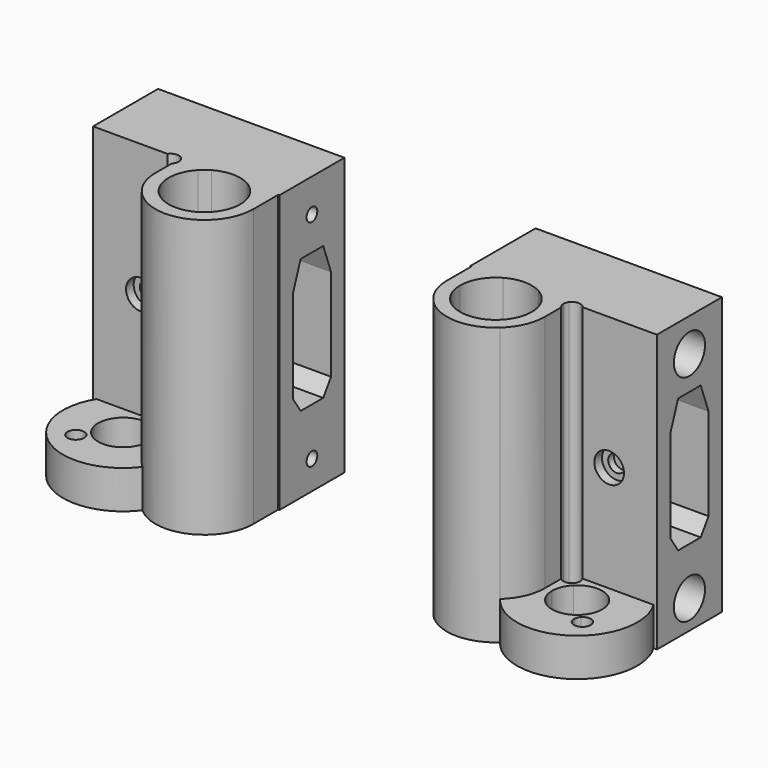
from build123d import *
from build123d import SkipClean  # not in build123d's __all__

# Parameters (mm, degrees)
F0_W           = 39
F0_H           = 58
F1_DEPTH       = 17
F3_DEPTH       = 58.001
F4_DEPTH       = 58
F5_DEPTH       = 8
F7_DEPTH       = 39.001
F6_R           = 4.075
F8_DEPTH       = 19.6
F10_R          = 1.4
F9_R           = 1.4
F11_DEPTH      = 19.401
F12_R          = 1.8
F13_DEPTH      = 3.501
F13_DEPTH_BACK = 32.601
F14_R          = 3.1
F14_R_2        = 1.8
F15_DEPTH      = 2
F16_R          = 1.8
F17_DEPTH      = 2


# Not quite as in the source:
# - a feature names something its author has since deleted; it is built from what else it names


with BuildPart() as f1:
    # F0 (on Front) → F1 (new body)
    with BuildSketch(Plane.XZ):
        with Locations((-21.25, -2)):
            Rectangle(F0_W, F0_H)
    extrude(amount=F1_DEPTH)

    # F2 (on face) → F3 (cut, through all)
    with BuildSketch(Plane(origin=(0, 0, -31), x_dir=(1, 0, 0), z_dir=(0, 0, -1))):
        with BuildLine():
            ThreePointArc((-15.9786113032, 17), (-12.25, 16.0065), (-8.5213886968, 17))
            Line((-8.5213886968, 17), (-15.9786113032, 17))
        make_face()
        with BuildLine():
            ThreePointArc((-25.186178146, 17), (-23.7501234559, 16.2501234559), (-22.3140687659, 17))
            Line((-22.3140687659, 17), (-22.5, 17))
            Line((-22.5, 17), (-25.186178146, 17))
        make_face()
        with BuildLine():
            Line((-22.5, 17), (-22.3140687659, 17))
            ThreePointArc((-22.3140687659, 17), (-22.0804534724, 17.4760031013), (-22.0001234559, 18.0001234559))
            ThreePointArc((-22.0001234559, 18.0001234559), (-22.1299049448, 18.6614796202), (-22.5, 19.2247423129))
            Line((-22.5, 19.2247423129), (-22.5, 17))
        make_face()
    extrude(amount=-F3_DEPTH, mode=Mode.SUBTRACT)

    # F2 (on face) → F4 (join, through all)
    with BuildSketch(Plane(origin=(0, 0, -31), x_dir=(1, 0, 0), z_dir=(0, 0, -1))):
        with BuildLine():
            ThreePointArc((-15.9786113032, 17), (-16.907616188, 17.6298080359), (-17.7321335956, 18.3913060876))
            ThreePointArc((-17.7321335956, 18.3913060876), (-18.0724084231, 17.6843790924), (-18.4560201964, 17))
            Line((-18.4560201964, 17), (-15.9786113032, 17))
        make_face()
        with BuildLine():
            ThreePointArc((-17.7321335956, 18.3913060876), (-19.7435, 23.5), (-17.7321335956, 28.6086939124))
            ThreePointArc((-17.7321335956, 28.6086939124), (-18.382014032, 29.8754906477), (-19.1706617647, 31.0608822725))
            ThreePointArc((-19.1706617647, 31.0608822725), (-21.6308124139, 27.6307212997), (-22.5, 23.5))
            Line((-22.5, 23.5), (-22.5, 19.2247423129))
            ThreePointArc((-22.5, 19.2247423129), (-22.1299049448, 18.6614796202), (-22.0001234559, 18.0001234559))
            ThreePointArc((-22.0001234559, 18.0001234559), (-22.0804534724, 17.4760031013), (-22.3140687659, 17))
            Line((-22.3140687659, 17), (-18.4560201964, 17))
            ThreePointArc((-18.4560201964, 17), (-18.0724084231, 17.6843790924), (-17.7321335956, 18.3913060876))
        make_face()
        with BuildLine():
            ThreePointArc((-17.7321335956, 28.6086939124), (-9.5048065504, 30.4725501199), (-4.7565, 23.5))
            ThreePointArc((-4.7565, 23.5), (-5.7656769416, 19.7441916017), (-8.5213886968, 17))
            Line((-8.5213886968, 17), (-2, 17))
            Line((-2, 17), (-2, 23.5))
            ThreePointArc((-2, 23.5), (-8.1192787003, 32.8808124139), (-19.1706617647, 31.0608822725))
            ThreePointArc((-19.1706617647, 31.0608822725), (-18.382014032, 29.8754906477), (-17.7321335956, 28.6086939124))
        make_face()
    with SkipClean():  # cleaning this boolean's faces spoils the solid; the shape is the same uncleaned
        extrude(amount=-F4_DEPTH)

    # F2 (on face) → F5 (join)
    with BuildSketch(Plane(origin=(0, 0, -31), x_dir=(1, 0, 0), z_dir=(0, 0, -1))):
        with BuildLine():
            ThreePointArc((-22.5, 23.5), (-21.6308124139, 27.6307212997), (-19.1706617647, 31.0608822725))
            ThreePointArc((-19.1706617647, 31.0608822725), (-36.289515659, 33.9501301086), (-40.0439798036, 17))
            Line((-40.0439798036, 17), (-25.186178146, 17))
            ThreePointArc((-25.186178146, 17), (-25.493269556, 18.1548544279), (-24.987560323, 19.237560323))
            ThreePointArc((-24.987560323, 19.237560323), (-23.7411060988, 19.7501002236), (-22.5, 19.2247423129))
            Line((-22.5, 19.2247423129), (-22.5, 23.5))
        make_face()
        with BuildLine():
            ThreePointArc((-24, 23.5), (-24.3996324543, 21.4909119801), (-25.5376893988, 19.7876893988))
            ThreePointArc((-25.5376893988, 19.7876893988), (-32.9623106012, 19.7876893988), (-32.9623106012, 27.2123106012))
            ThreePointArc((-32.9623106012, 27.2123106012), (-27.2409119801, 28.3503675457), (-24, 23.5))
        make_face(mode=Mode.SUBTRACT)
        with BuildLine():
            ThreePointArc((-32.9998765441, 28.9998765441), (-33.1330873622, 28.3301805374), (-33.512439677, 27.762439677))
            ThreePointArc((-33.512439677, 27.762439677), (-36.366665726, 29.6695725507), (-32.9998765441, 28.9998765441))
        make_face(mode=Mode.SUBTRACT)
    extrude(amount=-F5_DEPTH)

    # F6 (on face) → F7 (cut, through all)
    with BuildSketch(Plane(origin=(-40.75, 0, 0), x_dir=(0, -1, 0), z_dir=(-1, 0, 0))):
        Polygon((11.4548, 13), (5.5452, 13), (3.5, 7.381), (3.5, -11.9289), (5.5452, -15), (11.4548, -15), (13.5, -11.9289), (13.5, 7.381), align=None)
    extrude(amount=-F7_DEPTH, mode=Mode.SUBTRACT)

    # F6 (on face) → F8 (cut)
    with BuildSketch(Plane(origin=(-40.75, 0, 0), x_dir=(0, -1, 0), z_dir=(-1, 0, 0))):
        with Locations((8.5, 20)):
            Circle(F6_R)
        with Locations((8.5, -25)):
            Circle(F6_R)
    extrude(amount=-F8_DEPTH, mode=Mode.SUBTRACT)

    # F10 (on face) + F9 (on face) → F11 (cut, through all)
    with BuildSketch(Plane(origin=(-21.15, 0, 0), x_dir=(0, -1, 0), z_dir=(-1, 0, 0))):
        with Locations((8.5, -25)):
            Circle(F10_R)
    with BuildSketch(Plane(origin=(-21.15, 0, 0), x_dir=(0, -1, 0), z_dir=(-1, 0, 0))):
        with Locations((8.5, 20)):
            Circle(F9_R)
    extrude(amount=-F11_DEPTH, mode=Mode.SUBTRACT)

    # F12 (on face) → F13 (cut, two sides)
    with BuildSketch(Plane.XZ.offset(3.5)) as f13_sk:
        with Locations((-30.75, -0.75)):
            Circle(F12_R)
    extrude(amount=-F13_DEPTH, mode=Mode.SUBTRACT)
    extrude(f13_sk.sketch, amount=F13_DEPTH_BACK, mode=Mode.SUBTRACT)

    # F14 (on face) → F15 (cut)
    with BuildSketch(Plane.XZ.offset(17)):
        with Locations((-30.75, -0.75)):
            Circle(F14_R)
        with Locations((-30.75, -0.75)):
            Circle(F14_R_2, mode=Mode.SUBTRACT)
    extrude(amount=-F15_DEPTH, mode=Mode.SUBTRACT)

    # F16 (on face) → F17 (cut)
    with BuildSketch(Plane(origin=(0, 0, 0), x_dir=(-1, 0, 0), z_dir=(0, 1, 0))):
        Polygon((33.9482447703, -0.6440264703), (32.2573466163, 2.0727479835), (29.059101846, 1.9667744538), (27.5517552297, -0.8559735297), (29.2426533837, -3.5727479835), (32.440898154, -3.4667744538), align=None)
        with Locations((30.75, -0.75)):
            Circle(F16_R, mode=Mode.SUBTRACT)
    extrude(amount=-F17_DEPTH, mode=Mode.SUBTRACT)


with BuildPart() as f18_1:
    # F18: instance of F1
    add(f1.part.mirror(Plane(origin=(-1.75, -8.5, -2.2785977407), x_dir=(0, 1, 0), z_dir=(1, 0, 0))), clean=False)


with BuildPart() as f18_1_1:
    # F19: moved
    add(f18_1.part.moved(Location((40, 0, 0))), clean=False)


solid = Compound([f1.part, f18_1_1.part])
